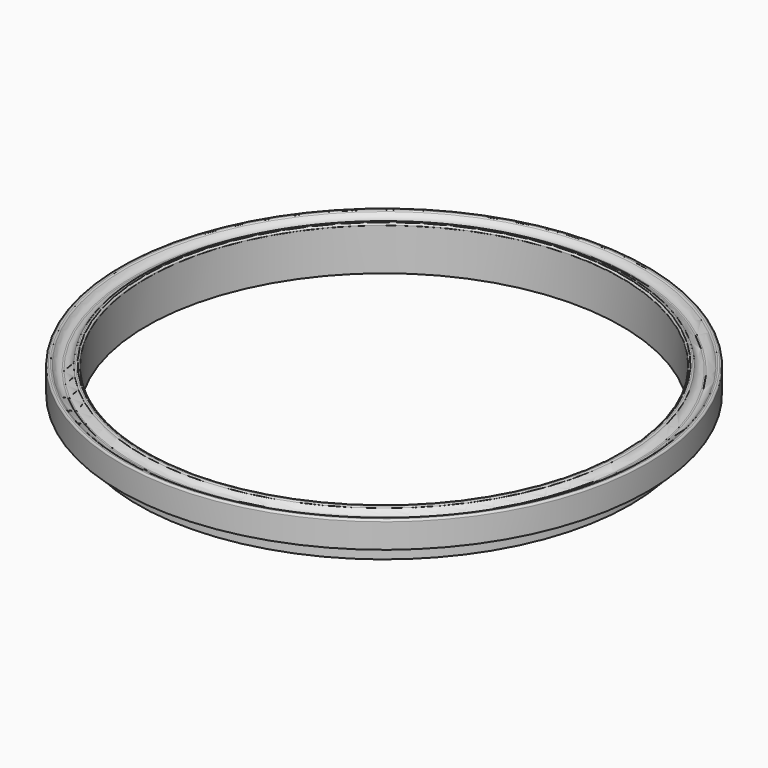
from build123d import *

# Parameters (mm, degrees)
F0_R     = 150
F0_R_2   = 135
F1_DEPTH = 25
F2_R     = 150
F2_R_2   = 140
F3_DEPTH = 10
F4_R     = 147.5
F4_R_2   = 137.5
F5_DEPTH = 3
F7_R     = 1
F8_R     = 1


# Not quite as in the source:
# - a fillet or chamfer that OpenCascade refuses, or shapes differently, is made with other operations: its cross-section is extruded or revolved along the edge and cut away or added


with BuildPart() as f1:
    # F0 (on Top) → F1 (new body)
    with BuildSketch(Plane.XY):
        Circle(F0_R)
        Circle(F0_R_2, mode=Mode.SUBTRACT)
    extrude(amount=F1_DEPTH)

    # F2 (on face) → F3 (cut)
    with BuildSketch(Plane(origin=(0, 0, 0), x_dir=(1, 0, 0), z_dir=(0, 0, -1))):
        Circle(F2_R)
        Circle(F2_R_2, mode=Mode.SUBTRACT)
    extrude(amount=-F3_DEPTH, mode=Mode.SUBTRACT)

    # F4 (on face) → F5 (cut)
    with BuildSketch(Plane.XY.offset(25)):
        Circle(F4_R)
        Circle(F4_R_2, mode=Mode.SUBTRACT)
    extrude(amount=-F5_DEPTH, mode=Mode.SUBTRACT)

    # F6: fillet of radius 5 on 2 edges, made by hand

    # F6_s1 → F6_t2 (revolve)
    with BuildSketch(Plane.XZ):
        with BuildLine():
            ThreePointArc((142.082575695, 22), (139.3439629074, 22.8166998673), (137.5, 25))
            Line((137.5, 25), (137.5, 22))
            Line((137.5, 22), (142.082575695, 22))
        make_face()
    revolve(axis=Axis((0, 0, 22), (0, 0, 1)))

    # F6_s3 → F6_t4 (revolve)
    with BuildSketch(Plane.XZ):
        with BuildLine():
            ThreePointArc((147.5, 25), (145.6560370926, 22.8166998673), (142.917424305, 22))
            Line((142.917424305, 22), (147.5, 22))
            Line((147.5, 22), (147.5, 25))
        make_face()
    revolve(axis=Axis((0, 0, 22), (0, 0, 1)))

    # F7
    f7_edges = [f1.edges().sort_by_distance(p)[0] for p in [
        (-147.5, 0, 25),
        (-150, 0, 25),
    ]]
    fillet(f7_edges, radius=F7_R)

    # F8
    f8_edges = [f1.edges().sort_by_distance(p)[0] for p in [
        (-137.5, 0, 25),
        (-135, 0, 25),
    ]]
    fillet(f8_edges, radius=F8_R)


solid = f1.part
